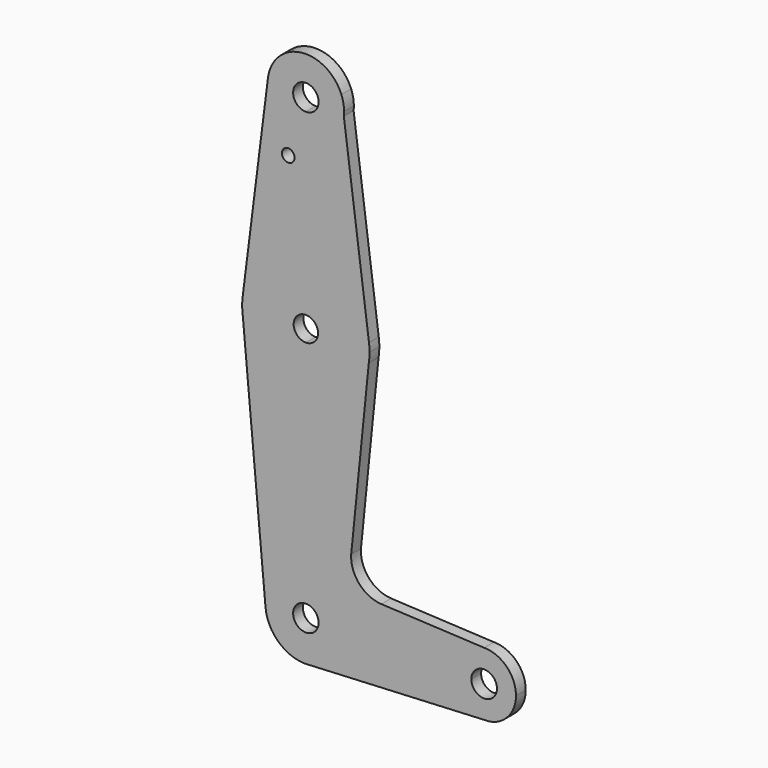
from build123d import *

# Parameters (mm, degrees)
F0_R     = 1.5875
F1_DEPTH = 3.048


# Not quite as in the source:
# - a feature names something its author has since deleted; it is built from what else it names


with BuildPart() as f1:
    # F0 (on Front) → F1 (new body)
    with BuildSketch(Plane.XZ):
        with BuildLine():
            Line((-35.5894761368, 60.4198244451), (-34.9866182967, 55.8428987828))
            ThreePointArc((-34.9866182967, 55.8428987828), (-34.9404170511, 56.3828619929), (-34.925, 56.9245788358))
            ThreePointArc((-34.925, 56.9245788358), (-35.092593447, 58.7035019936), (-35.5894761368, 60.4198244451))
        make_face()
        with BuildLine():
            Line((-60.2004882138, 4.1402033601), (-60.2004882138, 8.1089543114))
            ThreePointArc((-60.2004882138, 8.1089543114), (-60.325, 6.1245788358), (-60.2004882138, 4.1402033601))
        make_face()
        with BuildLine():
            ThreePointArc((-34.9866182967, 55.8428987828), (-38.1087610636, 49.8172365933), (-44.45, 47.3995788358))
            Line((-44.45, 47.3995788358), (-44.45, 21.9995788358))
            ThreePointArc((-44.45, 21.9995788358), (-33.9832619763, 18.0603662058), (-28.7109436839, 8.1976758617))
            Line((-28.7109436839, 8.1976758617), (-34.9866182967, 55.8428987828))
        make_face()
        with BuildLine():
            ThreePointArc((-44.45, -9.7504211642), (-54.950325336, -5.7816713228), (-60.2004882138, 4.1402033601))
            Line((-60.2004882138, 4.1402033601), (-54.5067664898, -58.2925744899))
            ThreePointArc((-54.5067664898, -58.2925744899), (-51.9079352447, -50.5666823428), (-44.45, -47.276920164))
            Line((-44.45, -47.276920164), (-44.45, -9.7504211642))
        make_face()
        with BuildLine():
            ThreePointArc((-34.3514989997, -57.3754211642), (-37.3092814629, -50.2347026271), (-44.45, -47.276920164))
            Line((-44.45, -47.276920164), (-44.45, -54.2004211642))
            ThreePointArc((-44.45, -54.2004211642), (-42.2049359697, -55.130357134), (-41.275, -57.3754211642))
            Line((-41.275, -57.3754211642), (-34.3514989997, -57.3754211642))
        make_face()
        with BuildLine():
            Line((-44.45, 21.9995788358), (-44.45, 47.3995788358))
            ThreePointArc((-44.45, 47.3995788358), (-51.5919689055, 50.6223645302), (-53.9009645367, 58.1098612184))
            Line((-53.9009645367, 58.1098612184), (-60.2004882138, 8.1089543114))
            ThreePointArc((-60.2004882138, 8.1089543114), (-54.950325336, 18.0308289943), (-44.45, 21.9995788358))
        make_face()
        with Locations((-48.8420496888, 42.732682374)):
            Circle(F0_R, mode=Mode.SUBTRACT)
        with BuildLine():
            ThreePointArc((-28.7109436839, 8.1976758617), (-33.9832619763, 18.0603662058), (-44.45, 21.9995788358))
            Line((-44.45, 21.9995788358), (-44.45, 9.1638046543))
            ThreePointArc((-44.45, 9.1638046543), (-42.3009428141, 8.2736360216), (-41.4107741814, 6.1245788358))
            ThreePointArc((-41.4107741814, 6.1245788358), (-42.3009428141, 3.9755216499), (-44.45, 3.0853530172))
            Line((-44.45, 3.0853530172), (-44.45, -9.7504211642))
            ThreePointArc((-44.45, -9.7504211642), (-34.1131196636, -5.9238455389), (-28.7595280627, 3.7111341226))
            ThreePointArc((-28.7595280627, 3.7111341226), (-28.6211992399, 4.91433444), (-28.575, 6.1245788358))
            ThreePointArc((-28.575, 6.1245788358), (-28.6090223784, 7.1633535905), (-28.7109436839, 8.1976758617))
        make_face()
        with BuildLine():
            ThreePointArc((-53.9009645367, 58.1098612184), (-51.5919689055, 50.6223645302), (-44.45, 47.3995788358))
            ThreePointArc((-44.45, 47.3995788358), (-38.1087610636, 49.8172365933), (-34.9866182967, 55.8428987828))
            Line((-34.9866182967, 55.8428987828), (-35.5894761368, 60.4198244451))
            ThreePointArc((-35.5894761368, 60.4198244451), (-45.6421147488, 66.37468399), (-53.9009645367, 58.1098612184))
        make_face()
        with BuildLine():
            ThreePointArc((-41.275, 56.9245788358), (-42.2049359697, 54.6795148055), (-44.45, 53.7495788358))
            ThreePointArc((-44.45, 53.7495788358), (-46.6950640303, 59.169642866), (-41.275, 56.9245788358))
        make_face(mode=Mode.SUBTRACT)
        with BuildLine():
            Line((-44.45, 9.1638046543), (-44.45, 21.9995788358))
            ThreePointArc((-44.45, 21.9995788358), (-54.950325336, 18.0308289943), (-60.2004882138, 8.1089543114))
            Line((-60.2004882138, 8.1089543114), (-60.2004882138, 4.1402033601))
            ThreePointArc((-60.2004882138, 4.1402033601), (-54.950325336, -5.7816713228), (-44.45, -9.7504211642))
            Line((-44.45, -9.7504211642), (-44.45, 3.0853530172))
            ThreePointArc((-44.45, 3.0853530172), (-47.4892258186, 6.1245788358), (-44.45, 9.1638046543))
        make_face()
        with BuildLine():
            Line((-7.9375, -57.3754211642), (-34.3514989997, -57.3754211642))
            ThreePointArc((-34.3514989997, -57.3754211642), (-36.803283354, -63.9714386739), (-42.9681138788, -67.3646021105))
            Line((-42.9681138788, -67.3646021105), (-0.5559922874, -65.2934246264))
            ThreePointArc((-0.5559922874, -65.2934246264), (-5.8059062614, -62.7879398695), (-7.9375, -57.3754211642))
        make_face()
        with BuildLine():
            ThreePointArc((-28.7595280627, 3.7111341226), (-34.1131196636, -5.9238455389), (-44.45, -9.7504211642))
            Line((-44.45, -9.7504211642), (-44.45, -47.276920164))
            ThreePointArc((-44.45, -47.276920164), (-37.3092814629, -50.2347026271), (-34.3514989997, -57.3754211642))
            Line((-34.3514989997, -57.3754211642), (-7.9375, -57.3754211642))
            ThreePointArc((-7.9375, -57.3754211642), (-5.6126600757, -51.7627610886), (0, -49.4379211642))
            Line((0, -49.4379211642), (-25.6033683849, -48.186229462))
            ThreePointArc((-25.6033683849, -48.186229462), (-31.1587660622, -45.5255963138), (-33.1463097303, -39.6954091582))
            Line((-33.1463097303, -39.6954091582), (-28.7595280627, 3.7111341226))
        make_face()
        with BuildLine():
            ThreePointArc((-44.45, -47.276920164), (-51.9079352447, -50.5666823428), (-54.5067664898, -58.2925744899))
            ThreePointArc((-54.5067664898, -58.2925744899), (-51.4418867888, -64.6619320978), (-44.9515214608, -67.4614609558))
            Line((-44.9515214608, -67.4614609558), (-42.9681138788, -67.3646021105))
            ThreePointArc((-42.9681138788, -67.3646021105), (-36.803283354, -63.9714386739), (-34.3514989997, -57.3754211642))
            Line((-34.3514989997, -57.3754211642), (-41.275, -57.3754211642))
            ThreePointArc((-41.275, -57.3754211642), (-46.6950640303, -59.6204851945), (-44.45, -54.2004211642))
            Line((-44.45, -54.2004211642), (-44.45, -47.276920164))
        make_face()
        with BuildLine():
            ThreePointArc((0, -49.4379211642), (-5.6126600757, -51.7627610886), (-7.9375, -57.3754211642))
            ThreePointArc((-7.9375, -57.3754211642), (-5.8059062614, -62.7879398695), (-0.5559922874, -65.2934246264))
            Line((-0.5559922874, -65.2934246264), (1.3248513243, -65.2015744479))
            ThreePointArc((1.3248513243, -65.2015744479), (6.0629989954, -62.4983060382), (7.9375, -57.3754211642))
            ThreePointArc((7.9375, -57.3754211642), (5.6126600757, -51.7627610886), (0, -49.4379211642))
        make_face()
        with BuildLine():
            ThreePointArc((3.1965151992, -57.3754211642), (0, -60.5719363635), (-3.1965151992, -57.3754211642))
            ThreePointArc((-3.1965151992, -57.3754211642), (0, -54.178905965), (3.1965151992, -57.3754211642))
        make_face(mode=Mode.SUBTRACT)
    extrude(amount=F1_DEPTH)


solid = f1.part
